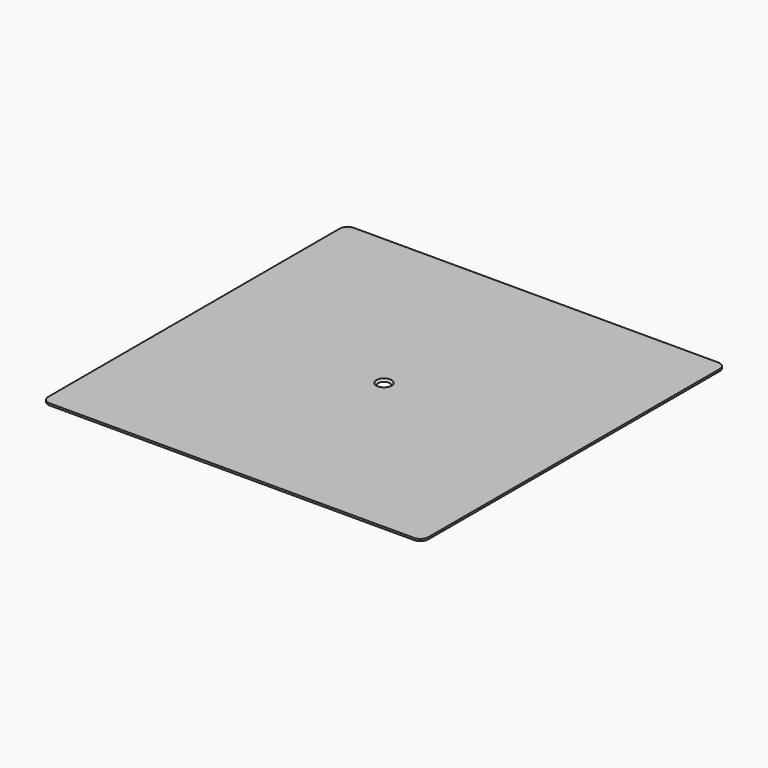
from build123d import *

# Parameters (mm, degrees)
F0_W           = 304.8
F0_H           = 304.8
F1_DEPTH       = 1.5875
F2_R           = 6.35
F4_D           = 6.2
F4_CSINK_D     = 12.2
F4_CSINK_ANGLE = 90


# Not quite as in the source:
# - a length typed as a fraction of an inch, garbled in the dataset ("3 / 203.2 mm" for 3/8 in), is restored


with BuildPart() as f1:
    # F0 (on Top) → F1 (new body)
    with BuildSketch(Plane.XY):
        Rectangle(F0_W, F0_H)
    extrude(amount=F1_DEPTH)

    # F2
    f2_edges = [f1.edges().sort_by_distance(p)[0] for p in [
        (-152.4, -152.4, 0.79375),
        (152.4, -152.4, 0.79375),
        (152.4, 152.4, 0.79375),
        (-152.4, 152.4, 0.79375),
    ]]
    fillet(f2_edges, radius=F2_R)

    # F4 (through all)
    with Locations(Plane.XY.offset(1.5875)):
        with Locations((0, 0)):
            CounterSinkHole(F4_D / 2, F4_CSINK_D / 2, counter_sink_angle=F4_CSINK_ANGLE)


solid = f1.part
